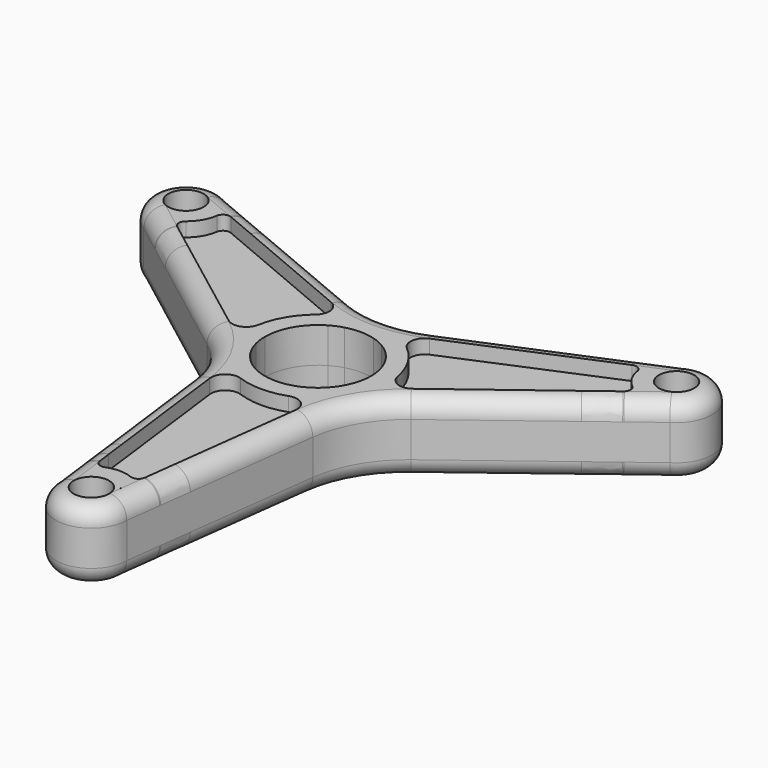
from build123d import *

# Parameters (mm, degrees)
F1_DEPTH = 6
F0_R     = 5
F2_DEPTH = 10
F3_R     = 4.99999


# Not quite as in the source:
# - a fillet or chamfer is up to 0.001 mm smaller than in the source, because OpenCascade refuses the exact size


with BuildPart() as f1:
    # F0 (on Top) → F1 (new body, symmetric)
    with BuildSketch(Plane.XY):
        with BuildLine():
            ThreePointArc((-3.650752169, -70.690219734), (0, -70), (3.650752169, -70.690219734))
            ThreePointArc((3.650752169, -70.690219734), (5.4029303192, -70.5474086273), (6.3654583562, -69.07633315))
            Line((6.3654583562, -69.07633315), (7.6770290576, -58.583767539))
            Line((7.6770290576, -58.583767539), (12.1161197255, -23.0710421958))
            ThreePointArc((12.1161197255, -23.0710421958), (10.6447389299, -19.4505887256), (6.7891735156, -18.8124193812))
            ThreePointArc((6.7891735156, -18.8124193812), (0, -20), (-6.7891735156, -18.8124193812))
            ThreePointArc((-6.7891735156, -18.8124193812), (-10.6447389299, -19.4505887256), (-12.1161197255, -23.0710421958))
            Line((-12.1161197255, -23.0710421958), (-6.8311160882, -65.3510712941))
            Line((-6.8311160882, -65.3510712941), (-6.3654583562, -69.07633315))
            ThreePointArc((-6.3654583562, -69.07633315), (-5.4029303192, -70.5474086273), (-3.650752169, -70.690219734))
        make_face()
    extrude(amount=F1_DEPTH, both=True)


with BuildPart() as f1b:
    # F0 (on Top) → F1, piece 2 (new body, symmetric)
    with BuildSketch(Plane.XY):
        with BuildLine():
            ThreePointArc((12.897446333, 15.2858064258), (15.3383874496, 12.8348693194), (17.3205080757, 10))
            ThreePointArc((17.3205080757, 10), (18.7845166096, 6.8659985248), (19.6866198486, 3.5266129555))
            ThreePointArc((19.6866198486, 3.5266129555), (22.1670734199, 0.5066800329), (26.0381684961, 1.0426536203))
            Line((26.0381684961, 1.0426536203), (63.0045884863, 29.0255179318))
            ThreePointArc((63.0045884863, 29.0255179318), (63.797313202, 30.5946294024), (63.0449021733, 32.1834657457))
            ThreePointArc((63.0449021733, 32.1834657457), (60.6217782649, 35), (59.3941500043, 38.5067539883))
            ThreePointArc((59.3941500043, 38.5067539883), (58.3943828828, 39.9527792249), (56.6391301301, 40.0508152183))
            Line((56.6391301301, 40.0508152183), (13.9220487706, 22.0283885755))
            ThreePointArc((13.9220487706, 22.0283885755), (11.52233449, 18.9439086927), (12.897446333, 15.2858064258))
        make_face()
    extrude(amount=F1_DEPTH, both=True)


with BuildPart() as f1c:
    # F0 (on Top) → F1, piece 3 (new body, symmetric)
    with BuildSketch(Plane.XY):
        with BuildLine():
            ThreePointArc((-59.3941500043, 38.5067539883), (-60.6217782649, 35), (-63.0449021733, 32.1834657457))
            ThreePointArc((-63.0449021733, 32.1834657457), (-63.797313202, 30.5946294024), (-63.0045884863, 29.0255179318))
            Line((-63.0045884863, 29.0255179318), (-26.0381684961, 1.0426536203))
            ThreePointArc((-26.0381684961, 1.0426536203), (-22.1670734199, 0.5066800329), (-19.6866198486, 3.5266129555))
            ThreePointArc((-19.6866198486, 3.5266129555), (-18.7845166096, 6.8659985248), (-17.3205080757, 10))
            ThreePointArc((-17.3205080757, 10), (-15.3383874496, 12.8348693194), (-12.897446333, 15.2858064258))
            ThreePointArc((-12.897446333, 15.2858064258), (-11.52233449, 18.9439086927), (-13.9220487706, 22.0283885755))
            Line((-13.9220487706, 22.0283885755), (-56.6391301301, 40.0508152183))
            ThreePointArc((-56.6391301301, 40.0508152183), (-58.3943828828, 39.9527792249), (-59.3941500043, 38.5067539883))
        make_face()
    extrude(amount=F1_DEPTH, both=True)


with BuildPart() as f2:
    # F0 (on Top) → F2 (new body, symmetric)
    with BuildSketch(Plane.XY):
        with BuildLine():
            Line((-17.1973713214, -23.3314984557), (-10, -80))
            ThreePointArc((-10, -80), (0, -90), (10, -80))
            Line((10, -80), (17.1973713214, -23.3314984557))
            ThreePointArc((17.1973713214, -23.3314984557), (20.9775310882, -12.1113832207), (28.8043560317, -3.2276112148))
            Line((28.8043560317, -3.2276112148), (74.2820323028, 31.3397459622))
            ThreePointArc((74.2820323028, 31.3397459622), (77.9422863406, 45), (64.2820323028, 48.6602540378))
            Line((64.2820323028, 48.6602540378), (11.6069847103, 26.5591096705))
            ThreePointArc((11.6069847103, 26.5591096705), (0, 24.2227664414), (-11.6069847103, 26.5591096705))
            Line((-11.6069847103, 26.5591096705), (-64.2820323028, 48.6602540378))
            ThreePointArc((-64.2820323028, 48.6602540378), (-77.9422863406, 45), (-74.2820323028, 31.3397459622))
            Line((-74.2820323028, 31.3397459622), (-28.8043560317, -3.2276112148))
            ThreePointArc((-28.8043560317, -3.2276112148), (-20.9775310882, -12.1113832207), (-17.1973713214, -23.3314984557))
        make_face()
        with Locations((0, -80)):
            Circle(F0_R, mode=Mode.SUBTRACT)
        with BuildLine():
            ThreePointArc((6.3654583562, -69.07633315), (5.4029303192, -70.5474086273), (3.650752169, -70.690219734))
            ThreePointArc((3.650752169, -70.690219734), (0, -70), (-3.650752169, -70.690219734))
            ThreePointArc((-3.650752169, -70.690219734), (-5.4029303192, -70.5474086273), (-6.3654583562, -69.07633315))
            Line((-6.3654583562, -69.07633315), (-6.8311160882, -65.3510712941))
            Line((-6.8311160882, -65.3510712941), (-12.1161197255, -23.0710421958))
            ThreePointArc((-12.1161197255, -23.0710421958), (-10.6447389299, -19.4505887256), (-6.7891735156, -18.8124193812))
            ThreePointArc((-6.7891735156, -18.8124193812), (0, -20), (6.7891735156, -18.8124193812))
            ThreePointArc((6.7891735156, -18.8124193812), (10.6447389299, -19.4505887256), (12.1161197255, -23.0710421958))
            Line((12.1161197255, -23.0710421958), (7.6770290576, -58.583767539))
            Line((7.6770290576, -58.583767539), (6.3654583562, -69.07633315))
        make_face(mode=Mode.SUBTRACT)
        with Locations((-69.2820323028, 40)):
            Circle(F0_R, mode=Mode.SUBTRACT)
        with BuildLine():
            ThreePointArc((-63.0045884863, 29.0255179318), (-63.797313202, 30.5946294024), (-63.0449021733, 32.1834657457))
            ThreePointArc((-63.0449021733, 32.1834657457), (-60.6217782649, 35), (-59.3941500043, 38.5067539883))
            ThreePointArc((-59.3941500043, 38.5067539883), (-58.3943828828, 39.9527792249), (-56.6391301301, 40.0508152183))
            Line((-56.6391301301, 40.0508152183), (-13.9220487706, 22.0283885755))
            ThreePointArc((-13.9220487706, 22.0283885755), (-11.52233449, 18.9439086927), (-12.897446333, 15.2858064258))
            ThreePointArc((-12.897446333, 15.2858064258), (-15.3383874496, 12.8348693194), (-17.3205080757, 10))
            ThreePointArc((-17.3205080757, 10), (-18.7845166096, 6.8659985248), (-19.6866198486, 3.5266129555))
            ThreePointArc((-19.6866198486, 3.5266129555), (-22.1670734199, 0.5066800329), (-26.0381684961, 1.0426536203))
            Line((-26.0381684961, 1.0426536203), (-63.0045884863, 29.0255179318))
        make_face(mode=Mode.SUBTRACT)
        with BuildLine():
            ThreePointArc((7.5, 12.9903810568), (12.9903810568, 7.5), (15, 0))
            ThreePointArc((15, 0), (14.8841681507, -1.8605210188), (14.5384615385, -3.6923076923))
            ThreePointArc((14.5384615385, -3.6923076923), (12.9903810568, -7.5), (10.4668630294, -10.7445231781))
            ThreePointArc((10.4668630294, -10.7445231781), (9.0533425419, -11.9598072233), (7.5, -12.9903810568))
            ThreePointArc((7.5, -12.9903810568), (0, -15), (-7.5, -12.9903810568))
            ThreePointArc((-7.5, -12.9903810568), (-9.0533425419, -11.9598072233), (-10.4668630294, -10.7445231781))
            ThreePointArc((-10.4668630294, -10.7445231781), (-12.9903810568, -7.5), (-14.5384615385, -3.6923076923))
            ThreePointArc((-14.5384615385, -3.6923076923), (-14.8841681507, -1.8605210188), (-15, 0))
            ThreePointArc((-15, 0), (-12.9903810568, 7.5), (-7.5, 12.9903810568))
            ThreePointArc((-7.5, 12.9903810568), (-5.8308256088, 13.8203282421), (-4.0715985091, 14.4368308704))
            ThreePointArc((-4.0715985091, 14.4368308704), (0, 15), (4.0715985091, 14.4368308704))
            ThreePointArc((4.0715985091, 14.4368308704), (5.8308256088, 13.8203282421), (7.5, 12.9903810568))
        make_face(mode=Mode.SUBTRACT)
        with BuildLine():
            ThreePointArc((19.6866198486, 3.5266129555), (18.7845166096, 6.8659985248), (17.3205080757, 10))
            ThreePointArc((17.3205080757, 10), (15.3383874496, 12.8348693194), (12.897446333, 15.2858064258))
            ThreePointArc((12.897446333, 15.2858064258), (11.52233449, 18.9439086927), (13.9220487706, 22.0283885755))
            Line((13.9220487706, 22.0283885755), (56.6391301301, 40.0508152183))
            ThreePointArc((56.6391301301, 40.0508152183), (58.3943828828, 39.9527792249), (59.3941500043, 38.5067539883))
            ThreePointArc((59.3941500043, 38.5067539883), (60.6217782649, 35), (63.0449021733, 32.1834657457))
            ThreePointArc((63.0449021733, 32.1834657457), (63.797313202, 30.5946294024), (63.0045884863, 29.0255179318))
            Line((63.0045884863, 29.0255179318), (26.0381684961, 1.0426536203))
            ThreePointArc((26.0381684961, 1.0426536203), (22.1670734199, 0.5066800329), (19.6866198486, 3.5266129555))
        make_face(mode=Mode.SUBTRACT)
        with Locations((69.2820323028, 40)):
            Circle(F0_R, mode=Mode.SUBTRACT)
    extrude(amount=F2_DEPTH, both=True)

    # F3 (radius 5 in the source; OpenCascade refuses exactly that, so slightly less here)
    f3_edges = [f2.edges().sort_by_distance(p)[0] for p in [
        (51.543194, 14.056067, 10),
        (20.977531, -12.111383, 10),
        (13.598686, -51.665749, 10),
        (0, -90, 10),
        (-13.598686, -51.665749, 10),
        (-77.942286, 45, 10),
        (-51.543194, 14.056067, 10),
        (-20.977531, -12.111383, 10),
        (-37.944509, 37.609682, 10),
        (77.942286, 45, 10),
        (-13.598686, -51.665749, -10),
        (-77.942286, 45, -10),
        (0, -90, -10),
        (13.598686, -51.665749, -10),
        (20.977531, -12.111383, -10),
        (51.543194, 14.056067, -10),
        (77.942286, 45, -10),
        (37.944509, 37.609682, -10),
        (0, 24.222766, -10),
    ]]
    fillet(f3_edges, radius=F3_R)


solid = Compound([f1.part, f1b.part, f1c.part, f2.part])
